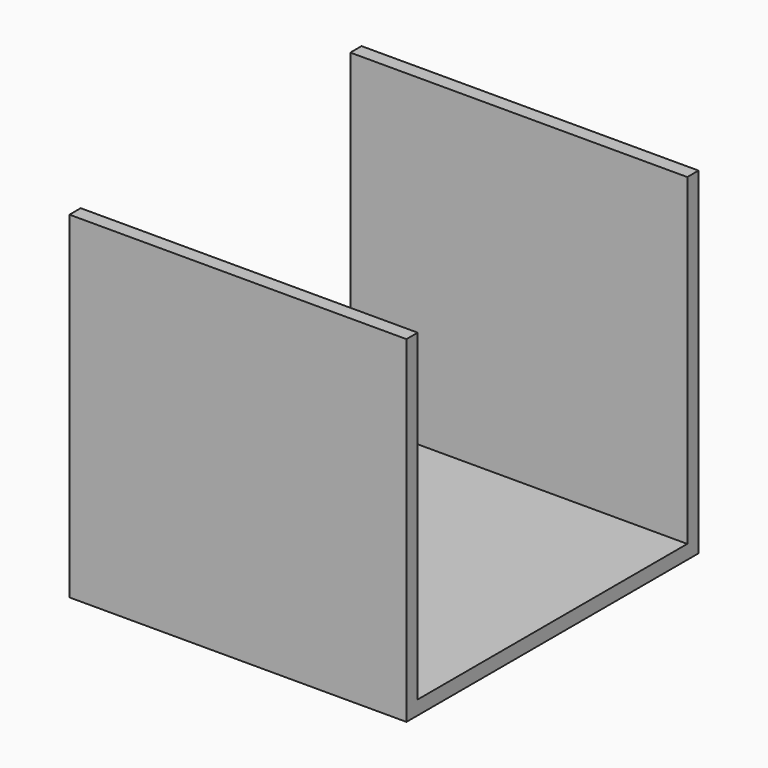
from build123d import *

# Parameters (mm, degrees)
F0_W     = 76.2
F0_H     = 76.2
F1_DEPTH = 3.175
F2_W     = 76.2
F2_H     = 73.025
F3_DEPTH = 3.175
F2_H_2   = 76.2
F4_DEPTH = 3.175
F5_W     = 76.2
F5_H     = 76.2
F6_DEPTH = 3.175


# Not quite as in the source:
# - a length typed as a fraction of an inch, garbled in the dataset ("3 / 203.2 mm" for 3/8 in), is restored


with BuildPart() as f1:
    # F0 (on Top) → F1 (new body)
    with BuildSketch(Plane.XY):
        Rectangle(F0_W, F0_H)
    extrude(amount=F1_DEPTH)

    # F2 (on face) → F3 (join)
    with BuildSketch(Plane.XZ.offset(38.1)):
        with Locations((0, 39.6875)):
            Rectangle(F2_W, F2_H)
    extrude(amount=F3_DEPTH)

    # F2 (on face) → F4 (join)
    with BuildSketch(Plane.XZ.offset(38.1)):
        with Locations((0, 38.1)):
            Rectangle(F2_W, F2_H_2)
    extrude(amount=F4_DEPTH)

    # F5 (on face) → F6 (join)
    with BuildSketch(Plane(origin=(0, 38.1, 0), x_dir=(-1, 0, 0), z_dir=(0, 1, 0))):
        with Locations((0, 38.1)):
            Rectangle(F5_W, F5_H)
    extrude(amount=F6_DEPTH)


solid = f1.part
